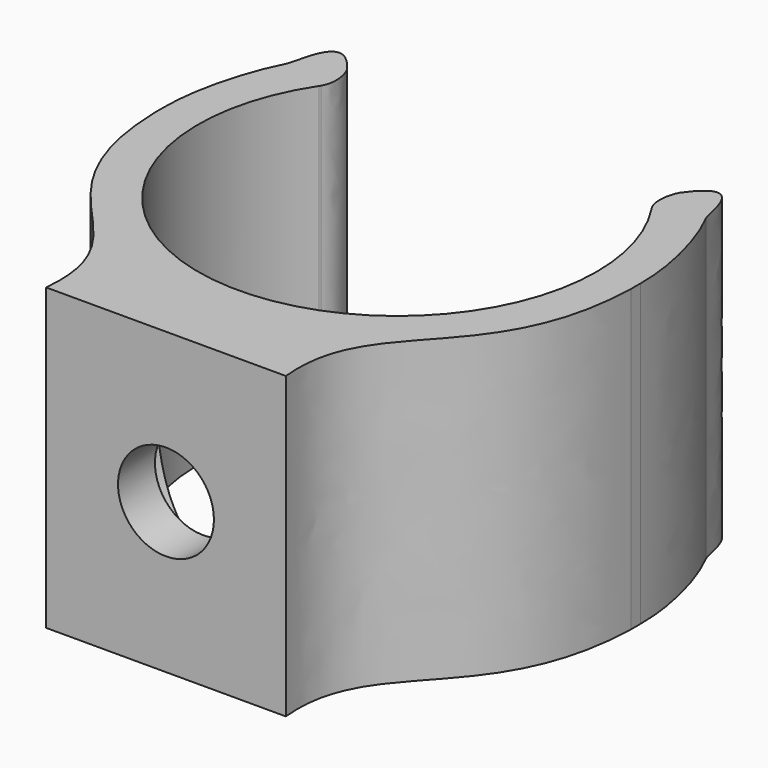
from build123d import *

# Parameters (mm, degrees)
F1_DEPTH = 10
F2_R     = 1.6
F3_DEPTH = 23.7
F2_R_2   = 3.5
F4_DEPTH = 8.11


with BuildPart() as f1:
    # F0 (on Top) → F1 (new body)
    with BuildSketch(Plane.XY):
        with BuildLine():
            ThreePointArc((5.55, 3.6633318168), (6.3690658656, 1.9124591499), (6.65, 0))
            ThreePointArc((6.65, 0), (-1.9124591499, -6.3690658656), (-5.55, 3.6633318168))
            ThreePointArc((-5.55, 3.6633318168), (-5.5352837539, 3.6855303232), (-5.5204787204, 3.7076697127))
            add(Edge.make_bspline(
                [(-5.5204787204, 3.7076697127), (-5.3297892382, 4.0203295099), (-5.3804192174, 4.5028316873), (-5.55, 4.8312691983)],
                knots=[0.0105120097, 0.0105120097, 0.0105120097, 0.0105120097, 0.2268448642, 0.2268448642, 0.2268448642, 0.2268448642], degree=3))
            add(Edge.make_bspline(
                [(-5.55, 4.8312691983), (-5.6230599396, 4.9344742738), (-5.6920586566, 5.0230662013), (-5.7572539606, 5.0984029712)],
                knots=[0, 0, 0, 0, 0.1009309198, 0.1009309198, 0.1009309198, 0.1009309198], degree=3))
            add(Edge.make_bspline(
                [(-5.7572539606, 5.0984029712), (-5.8127692495, 5.1426175603), (-6.1763134647, 5.3226921748), (-6.6399504917, 4.8081685915), (-6.9900612717, 4.1319315673)],
                knots=[0.2997379692, 0.2997379692, 0.2997379692, 0.2997379692, 0.350659585, 0.6091967522, 0.6091967522, 0.6091967522, 0.6091967522], degree=3))
            add(Edge.make_bspline(
                [(-6.9900612717, 4.1319315673), (-7.5192866492, 3.1097356941), (-7.9634342646, 1.5245852987), (-7.952605829, 0.2)],
                knots=[0.6091967522, 0.6091967522, 0.6091967522, 0.6091967522, 1, 1, 1, 1], degree=3))
            Line((-7.952605829, 0.2), (-7.952605829, 0))
            Line((-7.952605829, 0), (-7.952605829, -0.2))
            add(Edge.make_bspline(
                [(-7.952605829, -0.2), (-7.7880043421, -5.9189782478), (-3.58719808, -5.5995097942), (-4, -9.65)],
                knots=[0, 0, 0, 0, 10.2433194248, 10.2433194248, 10.2433194248, 10.2433194248], degree=3))
            Line((-4, -9.65), (0, -9.65))
            Line((0, -9.65), (4, -9.65))
            add(Edge.make_bspline(
                [(7.952605829, -0.2), (7.7880043421, -5.9189782478), (3.58719808, -5.5995097942), (4, -9.65)],
                knots=[0, 0, 0, 0, 10.2433194248, 10.2433194248, 10.2433194248, 10.2433194248], degree=3))
            Line((7.952605829, -0.2), (7.952605829, 0))
            Line((7.952605829, 0), (7.952605829, 0.2))
            add(Edge.make_bspline(
                [(6.9900612717, 4.1319315673), (7.5192866492, 3.1097356941), (7.9634342646, 1.5245852987), (7.952605829, 0.2)],
                knots=[0.6091967522, 0.6091967522, 0.6091967522, 0.6091967522, 1, 1, 1, 1], degree=3))
            add(Edge.make_bspline(
                [(5.7572539606, 5.0984029712), (5.8127692495, 5.1426175603), (6.1763134647, 5.3226921748), (6.6399504917, 4.8081685915), (6.9900612717, 4.1319315673)],
                knots=[0.2997379692, 0.2997379692, 0.2997379692, 0.2997379692, 0.350659585, 0.6091967522, 0.6091967522, 0.6091967522, 0.6091967522], degree=3))
            add(Edge.make_bspline(
                [(5.55, 4.8312691983), (5.6230599396, 4.9344742738), (5.6920586566, 5.0230662013), (5.7572539606, 5.0984029712)],
                knots=[0, 0, 0, 0, 0.1009309198, 0.1009309198, 0.1009309198, 0.1009309198], degree=3))
            add(Edge.make_bspline(
                [(5.5204787204, 3.7076697127), (5.3297892382, 4.0203295099), (5.3804192174, 4.5028316873), (5.55, 4.8312691983)],
                knots=[0.0105120097, 0.0105120097, 0.0105120097, 0.0105120097, 0.2268448642, 0.2268448642, 0.2268448642, 0.2268448642], degree=3))
            ThreePointArc((5.5204787204, 3.7076697127), (5.5352837539, 3.6855303232), (5.55, 3.6633318168))
        make_face()
        with BuildLine():
            add(Edge.make_bspline(
                [(5.7572539606, 5.0984029712), (6.726137476, 6.2180013153), (6.8550118896, 4.4101097728), (6.9900612717, 4.1319315673)],
                knots=[0.1009309198, 0.1009309198, 0.1009309198, 0.1009309198, 1.6008902487, 1.6008902487, 1.6008902487, 1.6008902487], degree=3))
            add(Edge.make_bspline(
                [(5.7572539606, 5.0984029712), (5.8127692495, 5.1426175603), (6.1763134647, 5.3226921748), (6.6399504917, 4.8081685915), (6.9900612717, 4.1319315673)],
                knots=[0.2997379692, 0.2997379692, 0.2997379692, 0.2997379692, 0.350659585, 0.6091967522, 0.6091967522, 0.6091967522, 0.6091967522], degree=3))
        make_face()
        with BuildLine():
            add(Edge.make_bspline(
                [(-5.7572539606, 5.0984029712), (-5.8127692495, 5.1426175603), (-6.1763134647, 5.3226921748), (-6.6399504917, 4.8081685915), (-6.9900612717, 4.1319315673)],
                knots=[0.2997379692, 0.2997379692, 0.2997379692, 0.2997379692, 0.350659585, 0.6091967522, 0.6091967522, 0.6091967522, 0.6091967522], degree=3))
            add(Edge.make_bspline(
                [(-5.7572539606, 5.0984029712), (-6.726137476, 6.2180013153), (-6.8550118896, 4.4101097728), (-6.9900612717, 4.1319315673)],
                knots=[0.1009309198, 0.1009309198, 0.1009309198, 0.1009309198, 1.6008902487, 1.6008902487, 1.6008902487, 1.6008902487], degree=3))
        make_face()
    extrude(amount=F1_DEPTH)

    # F2 (on Front) → F3 (cut)
    with BuildSketch(Plane.XZ):
        with Locations((0, 5)):
            Circle(F2_R)
    extrude(amount=F3_DEPTH, mode=Mode.SUBTRACT)

    # F2 (on Front) → F4 (cut)
    with BuildSketch(Plane.XZ):
        with Locations((0, 5)):
            Circle(F2_R_2)
        with Locations((0, 5)):
            Circle(F2_R, mode=Mode.SUBTRACT)
    extrude(amount=F4_DEPTH, mode=Mode.SUBTRACT)


solid = f1.part
